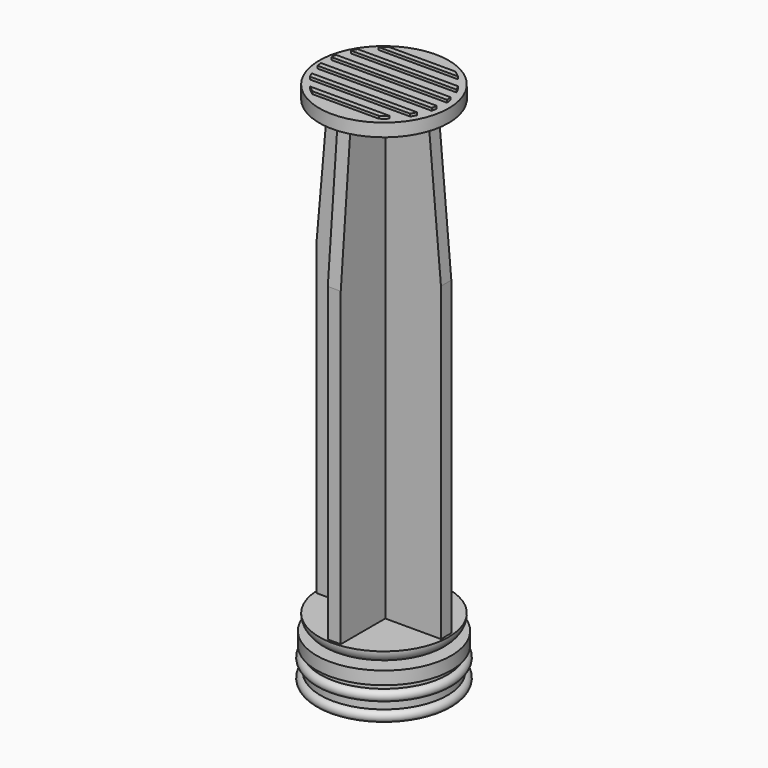
from build123d import *

# Parameters (mm, degrees)
F0_R      = 25
F1_DEPTH  = 5
F3_DEPTH  = 2.5
F5_DEPTH  = 2.5
F6_R      = 25
F7_DEPTH  = 5
F10_R     = 4.99999
F12_DEPTH = 1


# Not quite as in the source:
# - a fillet or chamfer is up to 0.001 mm smaller than in the source, because OpenCascade refuses the exact size


with BuildPart() as f1:
    # F0 (on Top) → F1 (new body)
    with BuildSketch(Plane.XY):
        Circle(F0_R)
    extrude(amount=F1_DEPTH)

    # F2 (on Front) → F3 (join, symmetric)
    with BuildSketch(Plane.XZ):
        Polygon((-24, 125), (-24, 5), (24, 5), (24, 125), (18.7706554351, 184.7716818855), (-18.7706554351, 184.7716818855), align=None)
    extrude(amount=F3_DEPTH, both=True)

    # F4 (on Right) → F5 (join, symmetric)
    with BuildSketch(Plane.YZ):
        Polygon((-24, 125), (-24, 5), (24, 5), (24, 125), (18.7706554351, 184.7716818855), (-18.7706554351, 184.7716818855), align=None)
    extrude(amount=F5_DEPTH, both=True)

    # F6 (on face) → F7 (join)
    with BuildSketch(Plane.XY.offset(184.7716818855)):
        Circle(F6_R)
        Polygon((-2.5, -2.5), (-18.7706554351, -2.5), (-18.7706554351, 2.5), (-2.5, 2.5), (-2.5, 18.7706554351), (2.5, 18.7706554351), (2.5, 2.5), (18.7706554351, 2.5), (18.7706554351, -2.5), (2.5, -2.5), (2.5, -18.7706554351), (-2.5, -18.7706554351), align=None, mode=Mode.SUBTRACT)
    extrude(amount=-F7_DEPTH)

    # F10 (radius 5 in the source; OpenCascade refuses exactly that, so slightly less here)
    f10_edges = [f1.edges().sort_by_distance(p)[0] for p in [
        (-25, 0, 0),
    ]]
    fillet(f10_edges, radius=F10_R)

    # F11 (on face) → F12 (join)
    with BuildSketch(Plane.XY.offset(184.7716818855)):
        with BuildLine():
            ThreePointArc((12.8062484749, -18.5), (14.0871915691, -17.5442592803), (15.2970585408, -16.5))
            Line((15.2970585408, -16.5), (-15.2970585408, -16.5))
            ThreePointArc((-15.2970585408, -16.5), (-14.0871915691, -17.5442592803), (-12.8062484749, -18.5))
            Line((-12.8062484749, -18.5), (12.8062484749, -18.5))
        make_face()
        with BuildLine():
            ThreePointArc((19.3390796058, -11.5), (19.8927295405, -10.5132921309), (20.3960780544, -9.5))
            Line((20.3960780544, -9.5), (-20.3960780544, -9.5))
            ThreePointArc((-20.3960780544, -9.5), (-19.8927295405, -10.5132921309), (-19.3390796058, -11.5))
            Line((-19.3390796058, -11.5), (19.3390796058, -11.5))
        make_face()
        with BuildLine():
            ThreePointArc((22.045407685, -4.5), (22.2255517564, -3.5035480763), (22.360679775, -2.5))
            Line((22.360679775, -2.5), (-22.360679775, -2.5))
            ThreePointArc((-22.360679775, -2.5), (-22.2255517564, -3.5035480763), (-22.045407685, -4.5))
            Line((-22.045407685, -4.5), (22.045407685, -4.5))
        make_face()
        with BuildLine():
            Line((-22.360679775, 2.5), (22.360679775, 2.5))
            ThreePointArc((22.360679775, 2.5), (22.2255517564, 3.5035480763), (22.045407685, 4.5))
            Line((22.045407685, 4.5), (-22.045407685, 4.5))
            ThreePointArc((-22.045407685, 4.5), (-22.2255517564, 3.5035480763), (-22.360679775, 2.5))
        make_face()
        with BuildLine():
            Line((-20.3960780544, 9.5), (20.3960780544, 9.5))
            ThreePointArc((20.3960780544, 9.5), (19.8927295405, 10.5132921309), (19.3390796058, 11.5))
            Line((19.3390796058, 11.5), (-19.3390796058, 11.5))
            ThreePointArc((-19.3390796058, 11.5), (-19.8927295405, 10.5132921309), (-20.3960780544, 9.5))
        make_face()
        with BuildLine():
            Line((-15.2970585408, 16.5), (15.2970585408, 16.5))
            ThreePointArc((15.2970585408, 16.5), (14.0871915691, 17.5442592803), (12.8062484749, 18.5))
            Line((12.8062484749, 18.5), (-12.8062484749, 18.5))
            ThreePointArc((-12.8062484749, 18.5), (-14.0871915691, 17.5442592803), (-15.2970585408, 16.5))
        make_face()
    extrude(amount=F12_DEPTH)


with BuildPart() as f9:
    # F8 (on Right) → F9 (revolve)
    with BuildSketch(Plane.YZ):
        with BuildLine():
            Line((0, -25), (0, 0))
            Line((0, 0), (-3.0396745298, 0))
            Line((-3.0396745298, 0), (-3.0396745298, -1))
            Line((-3.0396745298, -1), (-26, -1))
            Line((-26, -1), (-26, -6))
            Line((-26, -6), (-24.5, -6))
            Line((-24.5, -6), (-24.5, -8))
            ThreePointArc((-24.5, -8), (-26.5, -10), (-24.5, -12))
            Line((-24.5, -12), (-24.5, -15))
            ThreePointArc((-24.5, -15), (-26.4858631671, -16.7626237555), (-24.9713967407, -18.9436525185))
            Line((-24.9713967407, -18.9436525185), (0, -25))
        make_face()
    revolve(axis=Axis((0, 0, -12.5), (0, 0, 1)))


solid = Compound([f1.part, f9.part])
